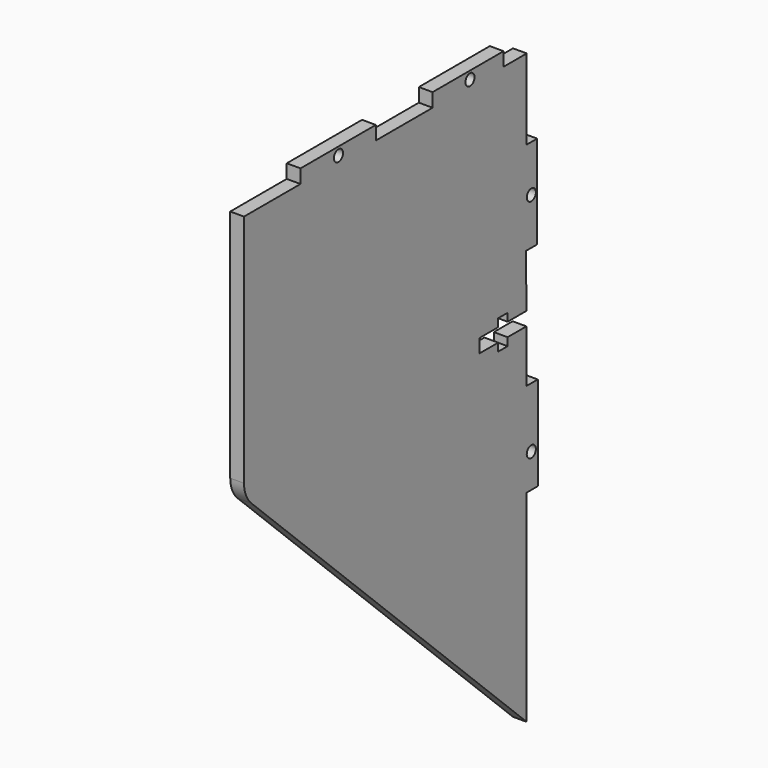
from build123d import *

# Parameters (mm, degrees)
F0_R     = 1.2331232955
F0_R_2   = 1.2314274958
F1_DEPTH = 2.9718


# Not quite as in the source:
# - a feature names something its author has since deleted; it is built from what else it names


with BuildPart() as f1:
    # F0 (on Right) → F1 (new body)
    with BuildSketch(Plane.YZ):
        with BuildLine():
            Line((-31.8963663923, 52.0706325769), (-31.8963663923, 69.3939922799))
            Line((-31.8963663923, 69.3939922799), (-36.9763663923, 69.3939922799))
            Line((-36.9763663923, 69.3939922799), (-38.147252053, 69.3939922799))
            Line((-38.147252053, 69.3939922799), (-38.147252053, 72.360080524))
            Line((-38.147252053, 72.360080524), (-57.2884293294, 72.360080524))
            Line((-57.2884293294, 72.360080524), (-57.2884293294, 69.3939922799))
            Line((-57.2884293294, 69.3939922799), (-72.6028546119, 69.3939922799))
            Line((-72.6028546119, 69.3939922799), (-72.6028546119, 72.360080524))
            Line((-72.6028546119, 72.360080524), (-92.9228546119, 72.360080524))
            Line((-92.9228546119, 72.360080524), (-92.9228546119, 69.3939922799))
            Line((-92.9228546119, 69.3939922799), (-108.1628546119, 69.3939922799))
            Line((-108.1628546119, 69.3939922799), (-108.1628546119, 18.7421012782))
            ThreePointArc((-108.1628546119, 18.7421012782), (-107.6580863604, 16.2610196982), (-106.2240307358, 14.1743857437))
            Line((-106.2240307358, 14.1743857437), (-31.8963663923, -57.6060077201))
            Line((-31.8963663923, -57.6060077201), (-31.8963663923, -16.9660077201))
            Line((-31.8963663923, -16.9660077201), (-31.8967170966, -14.0375348575))
            Line((-31.8967170966, -14.0375348575), (-28.9245663923, -14.0371789226))
            Line((-28.9245663923, -14.0371789226), (-28.9245663923, 3.3539922799))
            Line((-28.9245663923, 3.3539922799), (-28.9245663923, 6.2467521057))
            Line((-28.9245663923, 6.2467521057), (-31.8963663923, 6.2467521057))
            Line((-31.8963663923, 6.2467521057), (-31.988988285, 17.581195007))
            Line((-31.988988285, 17.581195007), (-37.0603909409, 17.581195007))
            Line((-37.0603909409, 17.581195007), (-37.0603909409, 15.8720928303))
            Line((-37.0603909409, 15.8720928303), (-39.6003909409, 15.8720928303))
            Line((-39.6003909409, 15.8720928303), (-39.6003909409, 17.581195007))
            Line((-39.6003909409, 17.581195007), (-44.6717935968, 17.581195007))
            Line((-44.6717935968, 17.581195007), (-44.6717935968, 20.5129906535))
            Line((-44.6717935968, 20.5129906535), (-39.6003909409, 20.5129906535))
            Line((-39.6003909409, 20.5129906535), (-39.6003909409, 22.2220928303))
            Line((-39.6003909409, 22.2220928303), (-37.0603909409, 22.2220928303))
            Line((-37.0603909409, 22.2220928303), (-37.0603909409, 20.5129906535))
            Line((-37.0603909409, 20.5129906535), (-31.988988285, 20.5129906535))
            Line((-31.988988285, 20.5129906535), (-32.0563334468, 28.7542376011))
            Line((-32.0563334468, 28.7542376011), (-32.0563334468, 31.9596784297))
            Line((-32.0563334468, 31.9596784297), (-29.0845334468, 31.9596784297))
            Line((-29.0845334468, 31.9596784297), (-29.0845334468, 49.0742376011))
            Line((-29.0845334468, 49.0742376011), (-29.0845334468, 52.0706325769))
            Line((-29.0845334468, 52.0706325769), (-31.8963663923, 52.0706325769))
        make_face()
        with Locations((-30.6644663923, -6.7510945896)):
            Circle(F0_R, mode=Mode.SUBTRACT)
        with Locations((-82.6862763941, 70.623036402)):
            Circle(F0_R_2, mode=Mode.SUBTRACT)
        with BuildLine():
            ThreePointArc((-29.4325663923, 42.0150328428), (-30.6644663923, 40.7831328428), (-31.8963663923, 42.0150328428))
            ThreePointArc((-31.8963663923, 42.0150328428), (-30.6644663923, 43.2469328428), (-29.4325663923, 42.0150328428))
        make_face(mode=Mode.SUBTRACT)
        with Locations((-47.2050075472, 70.623036402)):
            Circle(F0_R_2, mode=Mode.SUBTRACT)
    extrude(amount=F1_DEPTH)


solid = f1.part
